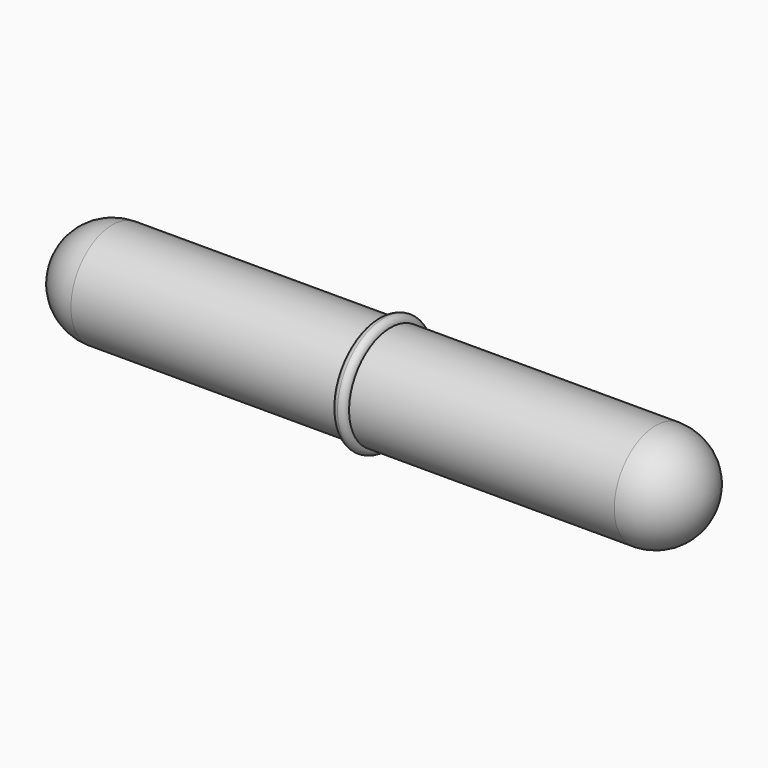
from build123d import *
from build123d import SkipClean  # not in build123d's __all__


with BuildPart() as f1:
    # F0 (on Top) → F1 (revolve)
    with BuildSketch(Plane.XY):
        with BuildLine():
            Line((0, 4), (0, 0))
            Line((0, 0), (21, 0))
            Line((21, 0), (25, 0))
            ThreePointArc((25, 0), (23.8284271247, 2.8284271247), (21, 4))
            Line((21, 4), (0.5, 4))
            Line((0.5, 4), (0, 4))
        make_face()
        with BuildLine():
            Line((0, 4.5), (0, 4))
            Line((0, 4), (0.5, 4))
            ThreePointArc((0.5, 4), (0.3535533906, 4.3535533906), (0, 4.5))
        make_face()
    revolve(axis=Axis((10.5, 0, 0), (1, 0, 0)))

    # F2: F1 across face


with BuildPart() as f1_1:
    add(f1.part, clean=False)
    with SkipClean():  # cleaning this boolean's faces spoils the solid; the shape is the same uncleaned
        add(f1.part.mirror(Plane(origin=(0, 0, 0), x_dir=(0, -1, 0), z_dir=(-1, 0, 0))), clean=False)


solid = f1_1.part
